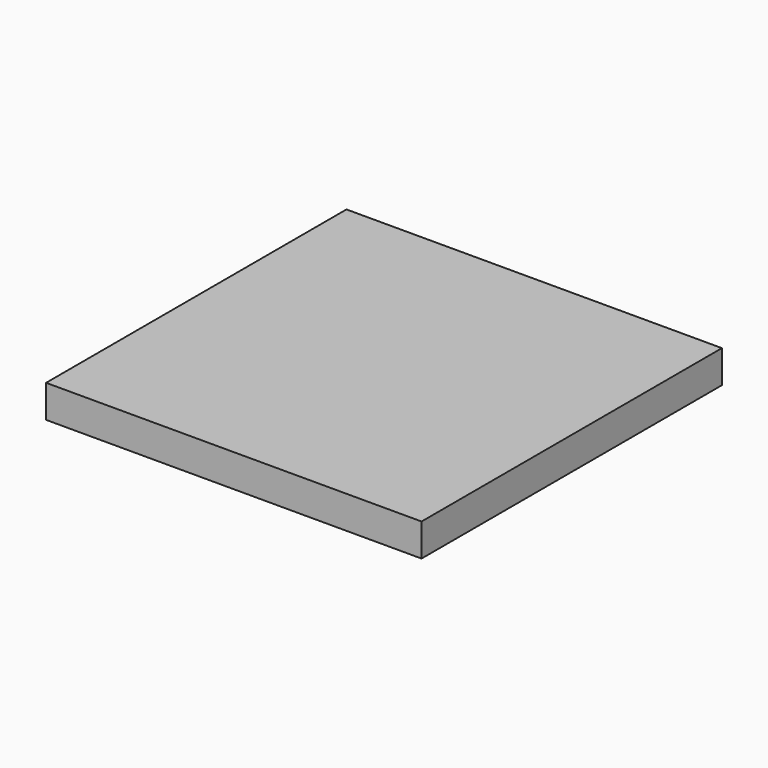
from build123d import *

# Parameters (mm, degrees)
F0_W     = 115
F0_H     = 115
F1_DEPTH = 10
F2_W     = 83
F2_H     = 62
F3_DEPTH = 6
F4_W     = 1
F4_H     = 62
F5_DEPTH = 6
F7_DEPTH = 8


# Not quite as in the source:
# - a feature of the source that left no trace in its solid (it failed there, or was rolled back) is left out


with BuildPart() as f1:
    # F0 (on Top) → F1 (new body)
    with BuildSketch(Plane.XY):
        Rectangle(F0_W, F0_H)
    extrude(amount=F1_DEPTH)

    # F2 (on face) → F3 (cut)
    with BuildSketch(Plane(origin=(0, 0, 0), x_dir=(1, 0, 0), z_dir=(0, 0, -1))):
        Rectangle(F2_W, F2_H)
    extrude(amount=-F3_DEPTH, mode=Mode.SUBTRACT)

    # F4 (on face) → F5 (join)
    with BuildSketch(Plane(origin=(0, 0, 0), x_dir=(1, 0, 0), z_dir=(0, 0, -1))):
        Rectangle(F4_W, F4_H)
    extrude(amount=-F5_DEPTH)

    # F6 (on face) → F7 (cut)
    with BuildSketch(Plane(origin=(0, 0, 0), x_dir=(1, 0, 0), z_dir=(0, 0, -1))):
        Polygon((-39.3114286867, 50.5), (-55.8729671482, 50.5), (-41.8729671482, 32), align=None)
        Polygon((-56.5, 33.1098824129), (-42.5, 31.1714208744), (-56.5, 49.6714208744), align=None)
        Polygon((-38.3018883964, 50.5), (-40.863426858, 32), (-24.3018883964, 32), align=None)
        Polygon((-20.4862842313, 50.5), (-37.0478226928, 50.5), (-23.0478226928, 32), align=None)
        Polygon((-19.4767439411, 50.5), (-22.0382824026, 32), (-5.4767439411, 32), align=None)
        Polygon((-1.0149211209, 50.5), (-18.2226782375, 50.5), (-4.2226782375, 32), align=None)
        Polygon((0, 50.5), (-3.2050376771, 32.0156837407), (3.2131379472, 32), align=None)
        Polygon((4.2226782375, 32), (18.2226782375, 50.5), (1.0149211209, 50.5), align=None)
        Polygon((22.0382824026, 32), (19.4767439411, 50.5), (5.4767439411, 32), align=None)
        Polygon((20.4862842313, 50.5), (23.0478226928, 32), (37.0478226928, 50.5), align=None)
        Polygon((40.863426858, 32), (38.3018883964, 50.5), (24.3018883964, 32), align=None)
        Polygon((39.3114286867, 50.5), (41.8729671482, 32), (55.8729671482, 50.5), align=None)
        Polygon((56.5, 49.6714208744), (42.5, 31.1714208744), (56.5, 33.1098824129), align=None)
        Polygon((-42.5, 13.6003421226), (-42.5, 30.1618805842), (-56.5, 32.1003421226), align=None)
        Polygon((-42.5, 11.9431838715), (-56.5, 30.4431838715), (-56.5, 13.8816454099), align=None)
        Polygon((-42.5, 1.2975080085), (-42.5, 10.9336435812), (-56.5, 12.8721051197), align=None)
        Polygon((-56.5, -13.8816454099), (-56.5, -30.4431838715), (-42.5, -11.9431838715), align=None)
        Polygon((-42.5, -13.6003421226), (-56.5, -32.1003421226), (-42.5, -30.1618805842), align=None)
        Polygon((-56.5, -49.6714208744), (-42.5, -31.1714208744), (-56.5, -33.1098824129), align=None)
        Polygon((-41.8729671482, -32), (-55.8729671482, -50.5), (-39.3114286867, -50.5), align=None)
        Polygon((56.5, 32.1003421226), (42.5, 30.1618805842), (42.5, 13.6003421226), align=None)
        Polygon((42.5, 11.9431838715), (56.5, 13.8816454099), (56.5, 30.4431838715), align=None)
        Polygon((56.5, -13.8816454099), (42.5, -11.9431838715), (56.5, -30.4431838715), align=None)
        Polygon((42.5, -30.1618805842), (56.5, -32.1003421226), (42.5, -13.6003421226), align=None)
        Polygon((56.5, -33.1098824129), (42.5, -31.1714208744), (56.5, -49.6714208744), align=None)
        Polygon((39.3114286867, -50.5), (55.8729671482, -50.5), (41.8729671482, -32), align=None)
        Polygon((-38.3018883964, -50.5), (-24.3018883964, -32), (-40.863426858, -32), align=None)
        Polygon((-23.0478226928, -32), (-37.0478226928, -50.5), (-20.4862842313, -50.5), align=None)
        Polygon((-5.4767439411, -32), (-22.0382824026, -32), (-19.4767439411, -50.5), align=None)
        Polygon((-4.2226782375, -32), (-18.2226782375, -50.5), (-1.0149211209, -50.5), align=None)
        Polygon((1.0149211209, -50.5), (18.2226782375, -50.5), (4.2226782375, -32), align=None)
        Polygon((5.4767439411, -32), (19.4767439411, -50.5), (22.0382824026, -32), align=None)
        Polygon((37.0478226928, -50.5), (23.0478226928, -32), (20.4862842313, -50.5), align=None)
        Polygon((24.3018883964, -32), (38.3018883964, -50.5), (40.863426858, -32), align=None)
        Polygon((3.2131379472, -32), (-3.2050376771, -32.0156837407), (0, -50.5), align=None)
        Polygon((56.5, 12.8721051197), (42.5, 10.9336435812), (42.5, 1.2975080085), align=None)
        Polygon((-42.5, 0), (-56.5, 11.5745971112), (-56.5, -11.5745971112), align=None)
        Polygon((56.5, -11.5745971112), (56.5, 11.5745971112), (42.5, 0), align=None)
        Polygon((-42.5, -10.9431838715), (-42.5, -1.2975080085), (-56.5, -12.8721051197), align=None)
        Polygon((42.5, -10.9431838715), (56.5, -12.8721051197), (42.5, -1.2975080085), align=None)
    extrude(amount=-F7_DEPTH, mode=Mode.SUBTRACT)


solid = f1.part
